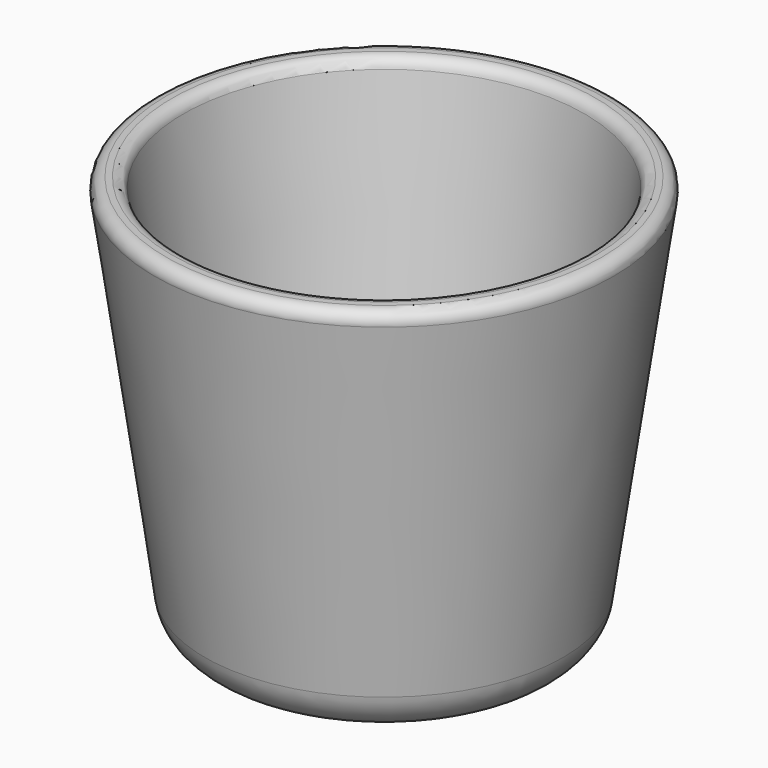
from build123d import *


# Not quite as in the source:
# - ends of sketch curves that miss each other by under 0.0002 mm in the source are joined


with BuildPart() as f1:
    # F0 (on Front) → F1 (revolve)
    with BuildSketch(Plane.XZ):
        with BuildLine():
            Line((0, 4.9999998882), (0, 0))
            Line((0, 0), (23.0616367864, 0))
            ThreePointArc((23.0616367864, 0), (28.3032507173, 1.95636836), (30.9812327357, 6.8686291501))
            Line((30.9812327357, 6.8686291501), (39.6738796125, 67.7171572875))
            ThreePointArc((39.6738796125, 67.7171572875), (39.2048885352, 69.3104034827), (37.6939806252, 70))
            Line((37.6939806252, 70), (36.6838267834, 70))
            ThreePointArc((36.6838267834, 70), (35.3734233007, 69.51090791), (34.7039277961, 68.2828427125))
            Line((34.7039277961, 68.2828427125), (26.0314839961, 7.5757361129))
            ThreePointArc((26.0314839961, 7.5757361129), (25.0272421924, 5.7336379253), (23.0616367864, 4.9999997224))
            Line((23.0616367864, 4.9999997224), (0, 4.9999998882))
        make_face()
    revolve(axis=Axis((0, 0, 2.4999999441), (0, 0, -1)))


solid = f1.part
